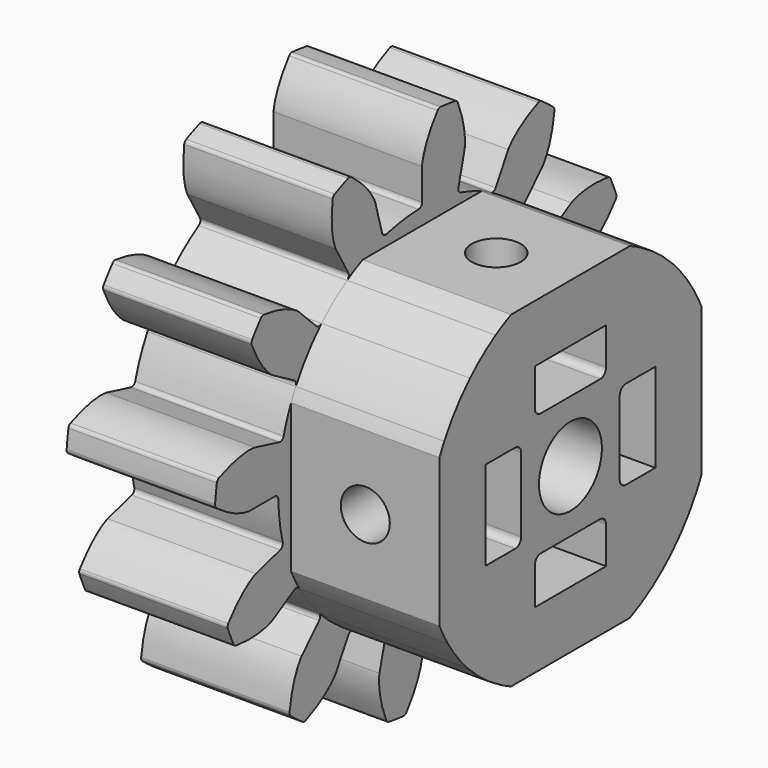
from build123d import *

# Parameters (mm, degrees)
F3_DEPTH        = 10
F3_COPIES_COUNT = 12
F4_R            = 0.3
F6_W            = 6
F6_H            = 3
F6_W_2          = 3
F6_H_2          = 6
F6_R            = 2.65
F7_DEPTH        = 10
F10_D           = 3.3
F10_ON_F8_D     = 3.3
F11_R           = 0.5
F12_DEPTH       = 10.0010001


# Not quite as in the source:
# - a feature of the source that left no trace in its solid (it failed there, or was rolled back) is left out
# - a pattern or mirror of a feature is missing from the dataset's text; its kind, count and spacing are read off the source's solid
# - a feature names something its author has since deleted; it is built from what else it names


with BuildPart() as f3:
    # F2 (on Right) → F3 (new body)
    with BuildSketch(Plane.YZ):
        with BuildLine():
            ThreePointArc((-12.1075, 0), (0, -12.1075), (12.1075, 0))
            ThreePointArc((12.1075, 0), (1.505491404, 12.0135361939), (-11.733103243, 2.9876151925))
            ThreePointArc((-11.733103243, 2.9876151925), (-12.0135361939, 1.505491404), (-12.1075, 0))
        make_face()
        with BuildLine():
            ThreePointArc((-12.1075, 0), (-12.0135361939, 1.505491404), (-11.733103243, 2.9876151925))
            Line((-11.733103243, 2.9876151925), (-14.0731483201, 3.5834638848))
            add(Edge.make_bspline(
                [(-17.2512872666, 2.9399128638), (-17.1861510595, 2.9695086261), (-16.9550530591, 3.0728407152), (-16.6410612871, 3.1939156286), (-16.2387708567, 3.3310174413), (-15.873495418, 3.4339391273), (-15.536823959, 3.5113538812), (-15.2329881244, 3.5652497599), (-14.962733076, 3.5993999505), (-14.7273855633, 3.617247847), (-14.5276450804, 3.62235704), (-14.3645320302, 3.6184435446), (-14.2370837845, 3.608825191), (-14.1492563767, 3.5981224941), (-14.091043051, 3.5874933402), (-14.0799612906, 3.5851986803), (-14.0731483201, 3.5834638848)],
                knots=[0.0628169841, 0.0628169841, 0.0628169841, 0.0628169841, 0.1050457383, 0.2061260475, 0.3030788746, 0.3957205093, 0.4838402817, 0.5671932426, 0.6454897173, 0.7183797703, 0.7854288699, 0.8460770668, 0.8995637563, 0.944768275, 0.9797835878, 1, 1, 1, 1], degree=3))
            ThreePointArc((-17.2512872666, 2.9399128638), (-17.3641861155, 2.1760148313), (-17.4432758959, 1.4078799729))
            add(Edge.make_bspline(
                [(-17.4432758959, 1.4078799729), (-17.3874568504, 1.3631265509), (-17.1890029848, 1.2059646293), (-16.914596821, 1.0111538882), (-16.558577189, 0.7790234959), (-16.2299937455, 0.5891500111), (-15.9228357449, 0.4310529583), (-15.6416945456, 0.3038499466), (-15.3882233288, 0.2040683401), (-15.1645575005, 0.1286986092), (-14.9722542665, 0.0744599645), (-14.8132194305, 0.0380030923), (-14.6873388305, 0.0158752228), (-14.599586315, 0.0045749006), (-14.5405502809, 0.0005108035), (-14.5292449743, 0), (-14.5222146057, 0)],
                knots=[0.0628169841, 0.0628169841, 0.0628169841, 0.0628169841, 0.1050457383, 0.2061260475, 0.3030788746, 0.3957205093, 0.4838402817, 0.5671932426, 0.6454897173, 0.7183797703, 0.7854288699, 0.8460770668, 0.8995637563, 0.944768275, 0.9797835878, 1, 1, 1, 1], degree=3))
            Line((-14.5222146057, 0), (-12.1075, 0))
        make_face()
    extrude(amount=F3_DEPTH)

    # F3_copies: F3 ×12 about axis
    f3_copies_axis = Axis((0, 0, 0), (1, 0, 0))


with BuildPart() as f3_1:
    add(f3.part)
    for i in range(1, F3_COPIES_COUNT):
        add(f3.part.rotate(f3_copies_axis, i * 360 / F3_COPIES_COUNT))

    # F4
    f4_edges = [f3_1.edges().sort_by_distance(p)[0] for p in [
        (5, -11.733103, 2.987615),
        (5, -17.251287, 2.939913),
        (5, -17.443276, 1.40788),
        (5, -12.1075, 0),
        (5, -11.654973, -3.279201),
        (5, 3.279201, -11.654973),
        (5, 0, -12.1075),
        (5, -2.987615, -11.733103),
        (5, -6.05375, -10.485403),
        (5, -8.453902, -8.667358),
        (5, -10.485403, -6.05375),
        (5, -10.485403, 6.05375),
        (5, -8.667358, 8.453902),
        (5, -6.05375, 10.485403),
        (5, -3.279201, 11.654973),
        (5, 0, 12.1075),
        (5, 2.987615, 11.733103),
        (5, 6.05375, 10.485403),
        (5, 8.453902, 8.667358),
        (5, 10.485403, 6.05375),
        (5, 11.654973, 3.279201),
        (5, 12.1075, 0),
        (5, 11.733103, -2.987615),
        (5, 10.485403, -6.05375),
        (5, 8.667358, -8.453902),
        (5, 6.05375, -10.485403),
        (5, -16.410009, -6.079604),
        (5, 7.502378, -15.81026),
        (5, 6.079604, -16.410009),
        (5, -1.40788, -17.443276),
        (5, -2.939913, -17.251287),
        (5, -9.940898, -14.40238),
        (5, -11.171683, -13.470097),
        (5, -15.81026, -7.502378),
        (5, -14.40238, 9.940898),
        (5, -13.470097, 11.171683),
        (5, -7.502378, 15.81026),
        (5, -6.079604, 16.410009),
        (5, 1.40788, 17.443276),
        (5, 2.939913, 17.251287),
        (5, 9.940898, 14.40238),
        (5, 11.171683, 13.470097),
        (5, 15.81026, 7.502378),
        (5, 16.410009, 6.079604),
        (5, 17.443276, -1.40788),
        (5, 17.251287, -2.939913),
        (5, 14.40238, -9.940898),
        (5, 13.470097, -11.171683),
    ]]
    fillet(f4_edges, radius=F4_R)

    # F6 (on face) → F7 (join)
    with BuildSketch(Plane.YZ.offset(10)):
        with BuildLine():
            ThreePointArc((10.6287102997, -5.7984544161), (10.835140598, -5.4028959338), (11.0268561363, -5))
            Line((11.0268561363, -5), (11.0268561363, 5))
            ThreePointArc((11.0268561363, 5), (10.7013367027, 5.6632984228), (10.3359639769, 6.3055059209))
            ThreePointArc((10.3359639769, 6.3055059209), (9.5593960895, 7.4303097279), (8.6609981397, 8.4604176891))
            ThreePointArc((8.6609981397, 8.4604176891), (7.310561898, 9.6512818312), (5.7984544161, 10.6287102997))
            ThreePointArc((5.7984544161, 10.6287102997), (5.4028959338, 10.835140598), (5, 11.0268561363))
            Line((5, 11.0268561363), (-5, 11.0268561363))
            ThreePointArc((-5, 11.0268561363), (-5.6632984228, 10.7013367027), (-6.3055059209, 10.3359639769))
            ThreePointArc((-6.3055059209, 10.3359639769), (-7.4303097279, 9.5593960895), (-8.4604176891, 8.6609981397))
            ThreePointArc((-8.4604176891, 8.6609981397), (-9.6512818312, 7.310561898), (-10.6287102997, 5.7984544161))
            ThreePointArc((-10.6287102997, 5.7984544161), (-10.835140598, 5.4028959338), (-11.0268561363, 5))
            Line((-11.0268561363, 5), (-11.0268561363, -5))
            ThreePointArc((-11.0268561363, -5), (-10.7013367027, -5.6632984228), (-10.3359639769, -6.3055059209))
            ThreePointArc((-10.3359639769, -6.3055059209), (-9.5593960895, -7.4303097279), (-8.6609981397, -8.4604176891))
            ThreePointArc((-8.6609981397, -8.4604176891), (-7.310561898, -9.6512818312), (-5.7984544161, -10.6287102997))
            ThreePointArc((-5.7984544161, -10.6287102997), (-5.4028959338, -10.835140598), (-5, -11.0268561363))
            Line((-5, -11.0268561363), (5, -11.0268561363))
            ThreePointArc((5, -11.0268561363), (5.6632984228, -10.7013367027), (6.3055059209, -10.3359639769))
            ThreePointArc((6.3055059209, -10.3359639769), (7.4303097279, -9.5593960895), (8.4604176891, -8.6609981397))
            ThreePointArc((8.4604176891, -8.6609981397), (9.6512818312, -7.310561898), (10.6287102997, -5.7984544161))
        make_face()
        with Locations((0, -5.65)):
            Rectangle(F6_W, F6_H, mode=Mode.SUBTRACT)
        with Locations((-5.65, 0)):
            Rectangle(F6_W_2, F6_H_2, mode=Mode.SUBTRACT)
        Circle(F6_R, mode=Mode.SUBTRACT)
        with Locations((5.65, 0)):
            Rectangle(F6_W_2, F6_H_2, mode=Mode.SUBTRACT)
        with Locations((0, 5.65)):
            Rectangle(F6_W, F6_H, mode=Mode.SUBTRACT)
    extrude(amount=F7_DEPTH)

    # F10 (through all)
    with Locations(Plane(origin=(0, 11.0268561363, 0), x_dir=(-1, 0, 0), z_dir=(0, 1, 0))):
        with Locations((-15, 0)):
            Hole(F10_D / 2)

    # F10 on F8 (through all)
    with Locations(Plane.XY.offset(11.0268561363)):
        with Locations((15, 0)):
            Hole(F10_ON_F8_D / 2)

    # F11
    f11_edges = [f3_1.edges().sort_by_distance(p)[0] for p in [
        (15, 4.15, -3),
        (15, 4.15, 3),
        (15, 3, -4.15),
        (15, -3, -4.15),
        (15, -3, 4.15),
        (15, 3, 4.15),
        (15, -4.15, -3),
        (15, -4.15, 3),
    ]]
    fillet(f11_edges, radius=F11_R)

    # F12 (cut, through all): a face of the model
    f12_faces = [f3_1.faces().sort_by_distance(p)[0] for p in [
        (10, 0, 0),
    ]]
    extrude(f12_faces, amount=-F12_DEPTH, mode=Mode.SUBTRACT)


solid = f3_1.part
